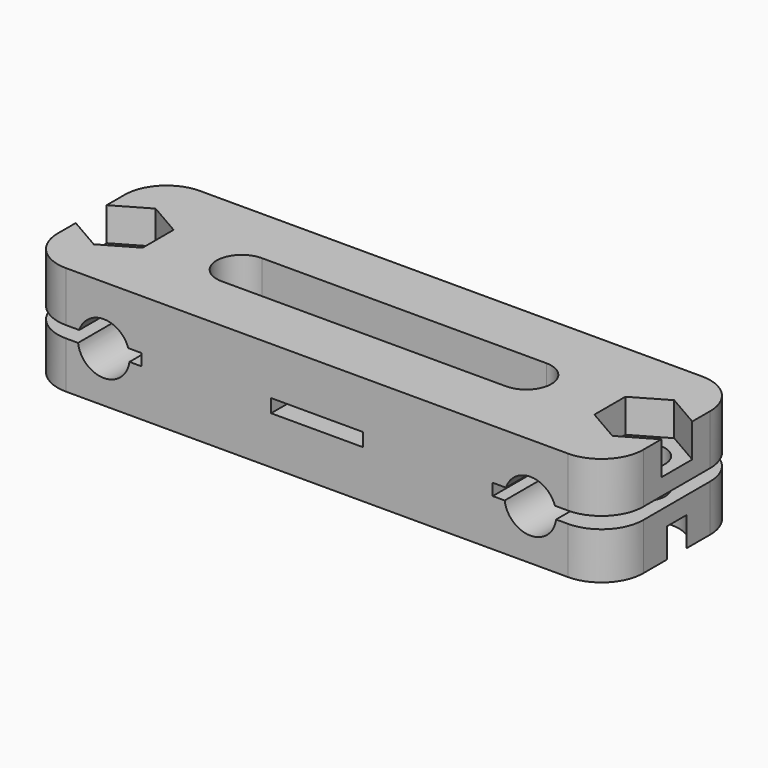
from build123d import *

# Parameters (mm, degrees)
F0_W      = 70
F0_H      = 20
F1_DEPTH  = 6.5
F4_DEPTH  = 4
F5_R      = 2.6
F6_DEPTH  = 13.001
F7_DEPTH  = 13.001
F9_R      = 5
F8_R      = 3.1
F10_DEPTH = 20.001
F11_W     = 45
F11_H     = 11
F12_DEPTH = 0.8
F13_W     = 11
F13_H     = 1.6
F14_DEPTH = 4.5
F15_W     = 14
F15_H     = 1.4
F16_DEPTH = 20.0010001
F17_R     = 4.25
F18_DEPTH = 3.5


with BuildPart() as f1:
    # F0 (on Top) → F1 (new body, symmetric)
    with BuildSketch(Plane.XY):
        Rectangle(F0_W, F0_H)
    extrude(amount=F1_DEPTH, both=True)

    # F3 (on face) → F4 (cut)
    with BuildSketch(Plane.XY.offset(6.5)):
        Polygon((-31, -4.6188021535), (-27, -2.3094010768), (-27, 2.3094010768), (-31, 4.6188021535), (-35, 2.3094010768), (-35, -2.3094010768), align=None)
        Polygon((35, -2.3094010768), (35, 2.3094010768), (31, 4.6188021535), (27, 2.3094010768), (27, -2.3094010768), (31, -4.6188021535), align=None)
    extrude(amount=-F4_DEPTH, mode=Mode.SUBTRACT)

    # F5 (on face) → F6 (cut, through all)
    with BuildSketch(Plane.XY.offset(6.5)):
        with Locations((-31, 0)):
            Circle(F5_R)
        with Locations((31, 0)):
            Circle(F5_R)
    extrude(amount=-F6_DEPTH, mode=Mode.SUBTRACT)

    # F2 (on face) → F7 (cut, through all)
    with BuildSketch(Plane.XY.offset(6.5)):
        with BuildLine():
            Line((-17, -3), (17, -3))
            ThreePointArc((17, -3), (20, 0), (17, 3))
            Line((17, 3), (-17, 3))
            ThreePointArc((-17, 3), (-20, 0), (-17, -3))
        make_face()
    extrude(amount=-F7_DEPTH, mode=Mode.SUBTRACT)

    # F9
    f9_edges = [f1.edges().sort_by_distance(p)[0] for p in [
        (35, -10, 0),
        (-35, -10, 0),
        (35, 10, 0),
        (-35, 10, 0),
    ]]
    fillet(f9_edges, radius=F9_R)

    # F8 (on face) → F10 (cut, through all)
    with BuildSketch(Plane.XZ.offset(10)):
        with Locations((-25.5, -0.5)):
            Circle(F8_R)
        with Locations((25.5, -0.5)):
            Circle(F8_R)
    extrude(amount=-F10_DEPTH, mode=Mode.SUBTRACT)

    # F11 (on Top) → F12 (cut, symmetric)
    with BuildSketch(Plane.XY):
        Rectangle(F11_W, F11_H)
    extrude(amount=F12_DEPTH, both=True, mode=Mode.SUBTRACT)

    # F13 (on face) → F14 (cut, through all)
    with BuildSketch(Plane.XZ.offset(10)):
        Rectangle(F13_W, F13_H)
    extrude(amount=-F14_DEPTH, mode=Mode.SUBTRACT)

    # F15 (on face) → F16 (cut, through all)
    with BuildSketch(Plane.XZ.offset(10)):
        with Locations((-28, -0.2)):
            Rectangle(F15_W, F15_H)
        with Locations((28, -0.2)):
            Rectangle(F15_W, F15_H)
    extrude(amount=-F16_DEPTH, mode=Mode.SUBTRACT)

    # F17 (on face) → F18 (cut)
    with BuildSketch(Plane(origin=(0, 0, -6.5), x_dir=(1, 0, 0), z_dir=(0, 0, -1))):
        with Locations((31, 0)):
            Circle(F17_R)
        with Locations((-31, 0)):
            Circle(F17_R)
    extrude(amount=-F18_DEPTH, mode=Mode.SUBTRACT)


solid = f1.part
